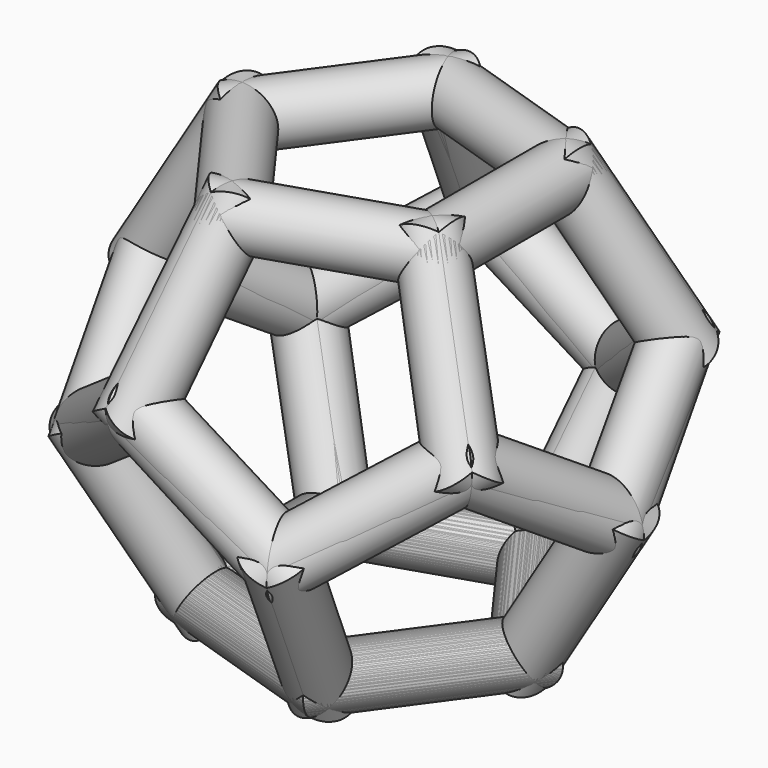
from build123d import *

# Parameters (mm, degrees)
F1_R     = 2.5
F3_ANGLE = 116
F5_COUNT = 5
F7_ANGLE = 36


with BuildPart() as f2:
    # F2: sweep along a path in F0
    with BuildLine(Plane.XY) as f2_path:
        Line((-9.7082039325, 7.0534230275), (-9.7082039325, -7.0534230275))
        Line((-9.7082039325, -7.0534230275), (3.7082039325, -11.4126781955))
        Line((3.7082039325, -11.4126781955), (12, 0))
        Line((12, 0), (3.7082039325, 11.4126781955))
        Line((3.7082039325, 11.4126781955), (-9.7082039325, 7.0534230275))
    # F1 (on Front) → F2 (sweep)
    with BuildSketch(Plane.XZ):
        with Locations((-9.7082039325, 0)):
            Circle(F1_R)
    sweep(path=f2_path.line, transition=Transition.RIGHT)


with BuildPart() as f3_1:
    # F3: copy of F2
    add(f2.part.rotate(Axis((-3, 9.2330506115, 0), (-0.9510565163, -0.3090169944, 0)), F3_ANGLE))


with BuildPart() as f5_1:
    # F5: instance of F3_1
    add(f3_1.part.rotate(Axis((0, 0, 16), (0, 0, 1)), 1 * 360 / F5_COUNT))


with BuildPart() as f5_2:
    # F5: instance of F3_1
    add(f3_1.part.rotate(Axis((0, 0, 16), (0, 0, 1)), 2 * 360 / F5_COUNT))


with BuildPart() as f5_3:
    # F5: instance of F3_1
    add(f3_1.part.rotate(Axis((0, 0, 16), (0, 0, 1)), 3 * 360 / F5_COUNT))


with BuildPart() as f5_4:
    # F5: instance of F3_1
    add(f3_1.part.rotate(Axis((0, 0, 16), (0, 0, 1)), 4 * 360 / F5_COUNT))


with BuildPart() as f6_1:
    # F6: instance of F2
    add(f2.part.mirror(Plane.XY))


with BuildPart() as f6_2:
    # F6: instance of F3_1
    add(f3_1.part.mirror(Plane.XY))


with BuildPart() as f6_3:
    # F6: instance of F5_2
    add(f5_2.part.mirror(Plane.XY))


with BuildPart() as f6_4:
    # F6: instance of F5_4
    add(f5_4.part.mirror(Plane.XY))


with BuildPart() as f6_5:
    # F6: instance of F5_3
    add(f5_3.part.mirror(Plane.XY))


with BuildPart() as f6_6:
    # F6: instance of F5_1
    add(f5_1.part.mirror(Plane.XY))


with BuildPart() as f6_4_1:
    # F7: moved
    add(f6_4.part.rotate(Axis((0, 0, 16), (0, 0, 1)), F7_ANGLE))


with BuildPart() as f6_5_1:
    # F7: moved
    add(f6_5.part.rotate(Axis((0, 0, 16), (0, 0, 1)), F7_ANGLE))


with BuildPart() as f6_3_1:
    # F7: moved
    add(f6_3.part.rotate(Axis((0, 0, 16), (0, 0, 1)), F7_ANGLE))


with BuildPart() as f6_6_1:
    # F7: moved
    add(f6_6.part.rotate(Axis((0, 0, 16), (0, 0, 1)), F7_ANGLE))


with BuildPart() as f6_2_1:
    # F7: moved
    add(f6_2.part.rotate(Axis((0, 0, 16), (0, 0, 1)), F7_ANGLE))


with BuildPart() as f6_4_2:
    # F8: moved
    add(f6_4_1.part.moved(Location((0, 0, 32))))


with BuildPart() as f6_5_2:
    # F8: moved
    add(f6_5_1.part.moved(Location((0, 0, 32))))


with BuildPart() as f6_3_2:
    # F8: moved
    add(f6_3_1.part.moved(Location((0, 0, 32))))


with BuildPart() as f6_6_2:
    # F8: moved
    add(f6_6_1.part.moved(Location((0, 0, 32))))


with BuildPart() as f6_2_2:
    # F8: moved
    add(f6_2_1.part.moved(Location((0, 0, 32))))


solid = Compound([f2.part, f3_1.part, f5_1.part, f5_2.part, f5_3.part, f5_4.part, f6_1.part, f6_4_2.part, f6_5_2.part, f6_3_2.part, f6_6_2.part, f6_2_2.part])
